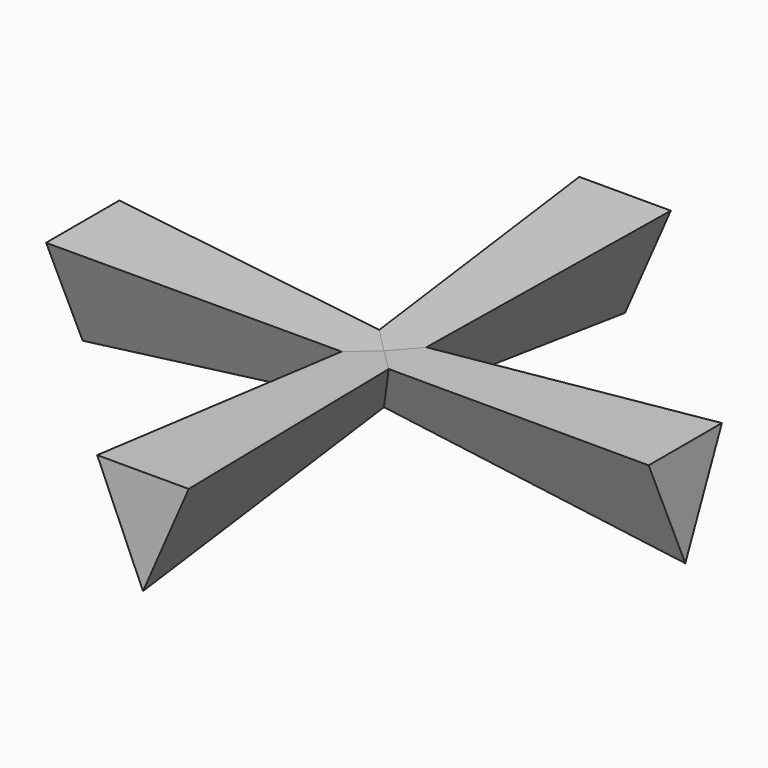
from build123d import *

# Parameters (mm, degrees)
F3_DEPTH        = 55.6593641
F3_TAPER        = -3
F3_COPIES_COUNT = 4


# Not quite as in the source:
# - an extrude ends at something that could not be found from the text; its depth is read off the source's solid
# - a feature of the source that left no trace in its solid (it failed there, or was rolled back) is left out
# - a pattern or mirror of a feature is missing from the dataset's text; its kind, count and spacing are read off the source's solid
# - the program builds the solid bodies; features that only make, move or delete a surface that nothing else refers to are left out


with BuildPart() as f3:
    # F2 (on Front) → F3 (new body, through all)
    with BuildSketch(Plane.XZ):
        Polygon((4, 28.3227710798), (0, 28.3227710798), (-4, 28.3227710798), (0, 19.1576196899), align=None)
    extrude(amount=-F3_DEPTH, taper=F3_TAPER)


with BuildPart() as f3_copies_1:
    # F3_copies: instance of F3
    add(f3.part.rotate(Axis((0, 0, 0), (0, 0, 1)), 1 * 360 / F3_COPIES_COUNT))


with BuildPart() as f3_copies_2:
    # F3_copies: instance of F3
    add(f3.part.rotate(Axis((0, 0, 0), (0, 0, 1)), 2 * 360 / F3_COPIES_COUNT))


with BuildPart() as f3_copies_3:
    # F3_copies: instance of F3
    add(f3.part.rotate(Axis((0, 0, 0), (0, 0, 1)), 3 * 360 / F3_COPIES_COUNT))


solid = Compound([f3.part, f3_copies_1.part, f3_copies_2.part, f3_copies_3.part])
